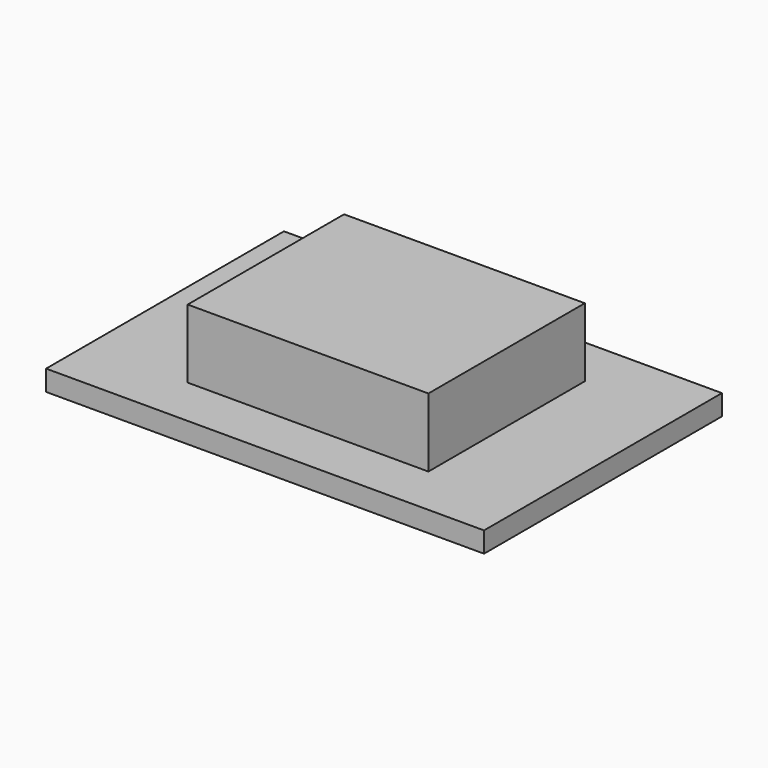
from build123d import *

# Parameters (mm, degrees)
F3_DEPTH = 5.842
F1_E1_W  = 68.4977713972
F1_E1_H  = 25.4
F4_DEPTH = 55.626


with BuildPart() as f3:
    # F2 (on Top) → F3 (new body)
    with BuildSketch(Plane.XY):
        Polygon((-66.1953240633, 37.8464572132), (-66.1953240633, 32.953761518), (-66.1953240633, -46.768438071), (51.8050417304, -46.768438071), (58.4245696664, -46.768438071), (58.4245696664, 37.8464572132), align=None)
    extrude(amount=F3_DEPTH)

    # F1_E1 (on explicit) → F4 (join)
    with BuildSketch(Plane(origin=(-37.4147482216, -32.3781482875, 0), x_dir=(1, 0, 0), z_dir=(0, -1, 0))):
        with Locations((34.2488856986, 12.7)):
            Rectangle(F1_E1_W, F1_E1_H)
    extrude(amount=-F4_DEPTH)


solid = f3.part
